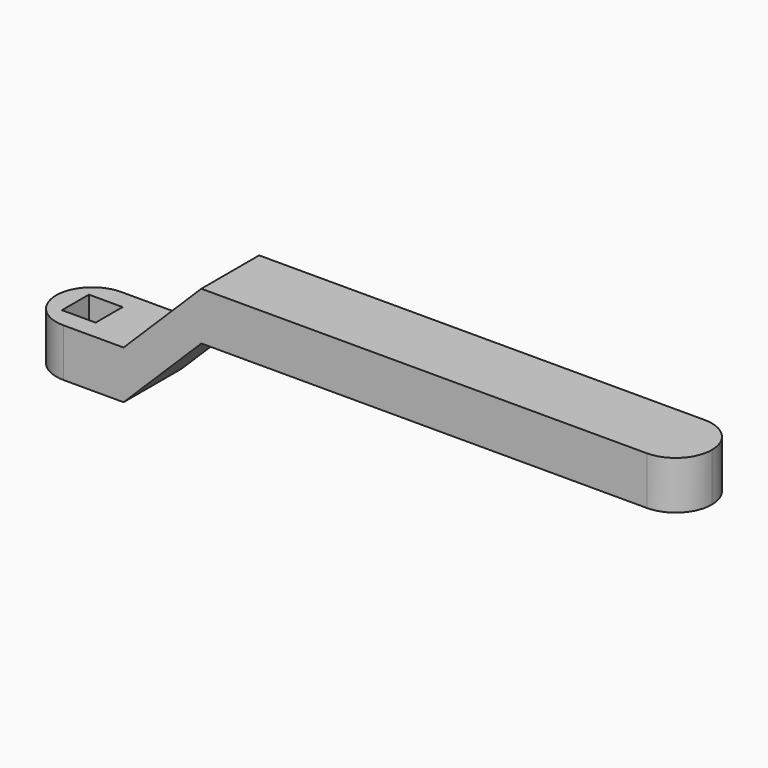
from build123d import *

# Parameters (mm, degrees)
F1_DEPTH      = 3.75
F1_DEPTH_BACK = 3.75
F2_W          = 3.5
F2_H          = 3.5
F3_DEPTH      = 5.001
F4_R          = 3.74999
F5_R          = 3.74999


# Not quite as in the source:
# - a fillet or chamfer is up to 0.001 mm smaller than in the source, because OpenCascade refuses the exact size


with BuildPart() as f1:
    # F0 (on Front) → F1 (new body, two sides)
    with BuildSketch(Plane.XZ) as f1_sk:
        Polygon((0, 5), (0, 0), (10, 0), (18.0723418804, 8), (68.0723418804, 8), (68.0723418804, 13), (18.0723418804, 13), (10, 5), align=None)
    extrude(amount=F1_DEPTH)
    extrude(f1_sk.sketch, amount=-F1_DEPTH_BACK)

    # F2 (on face) → F3 (cut, through all)
    with BuildSketch(Plane.XY.offset(5)):
        with Locations((3.75, 0)):
            Rectangle(F2_W, F2_H)
    extrude(amount=-F3_DEPTH, mode=Mode.SUBTRACT)

    # F4 (radius 3.75 in the source; OpenCascade refuses exactly that, so slightly less here)
    f4_edges = [f1.edges().sort_by_distance(p)[0] for p in [
        (0, -3.75, 2.5),
        (0, 3.75, 2.5),
    ]]
    fillet(f4_edges, radius=F4_R)

    # F5 (radius 3.75 in the source; OpenCascade refuses exactly that, so slightly less here)
    f5_edges = [f1.edges().sort_by_distance(p)[0] for p in [
        (68.072342, -3.75, 10.5),
        (68.072342, 3.75, 10.5),
    ]]
    fillet(f5_edges, radius=F5_R)


solid = f1.part
